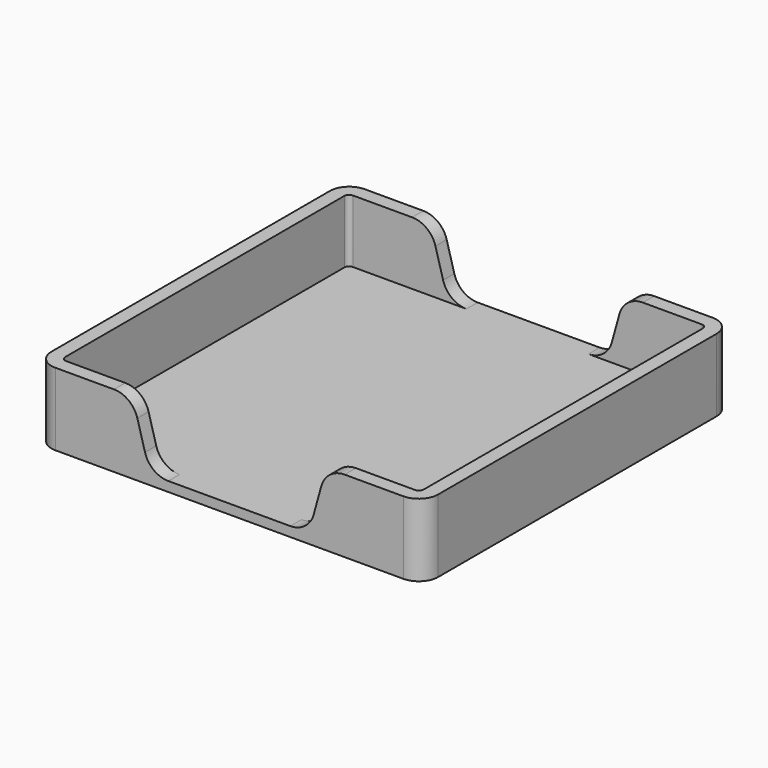
from build123d import *

# Parameters (mm, degrees)
F0_W      = 79.8
F0_H      = 79.8
F1_DEPTH  = 15
F2_W      = 74
F2_H      = 74
F3_DEPTH  = 13
F4_W      = 73.8
F4_H      = 73.8
F4_W_2    = 69.8
F4_H_2    = 69.8
F5_DEPTH  = 2
F7_DEPTH  = 2
F8_R      = 2
F9_R      = 4
F10_R     = 0.99999
F12_DEPTH = 79.801
F13_R     = 5
F14_R     = 4
F15_R     = 1


# Not quite as in the source:
# - a fillet or chamfer is up to 0.001 mm smaller than in the source, because OpenCascade refuses the exact size


with BuildPart() as f1:
    # F0 (on Top) → F1 (new body)
    with BuildSketch(Plane.XY):
        Rectangle(F0_W, F0_H)
    extrude(amount=F1_DEPTH)

    # F2 (on face) → F3 (cut)
    with BuildSketch(Plane.XY.offset(15)):
        Rectangle(F2_W, F2_H)
    extrude(amount=-F3_DEPTH, mode=Mode.SUBTRACT)

    # F4 (on face) → F5 (join)
    with BuildSketch(Plane(origin=(0, 0, 0), x_dir=(1, 0, 0), z_dir=(0, 0, -1))):
        Rectangle(F4_W, F4_H)
        Rectangle(F4_W_2, F4_H_2, mode=Mode.SUBTRACT)
    extrude(amount=F5_DEPTH)

    # F6 (on face) → F7 (cut, through all)
    with BuildSketch(Plane(origin=(0, 0, -2), x_dir=(1, 0, 0), z_dir=(0, 0, -1))):
        Polygon((36.9, -21.9), (36.9, 21.9), (21.9, 21.9), (21.9, 36.9), (-21.9, 36.9), (-21.9, 21.9), (-36.9, 21.9), (-36.9, -21.9), (-21.9, -21.9), (-21.9, -36.9), (21.9, -36.9), (21.9, -21.9), align=None)
    extrude(amount=-F7_DEPTH, mode=Mode.SUBTRACT)

    # F8
    f8_edges = [f1.edges().sort_by_distance(p)[0] for p in [
        (-34.9, 34.9, -1),
        (-34.9, -34.9, -1),
        (34.9, -34.9, -1),
        (34.9, 34.9, -1),
    ]]
    fillet(f8_edges, radius=F8_R)

    # F9
    f9_edges = [f1.edges().sort_by_distance(p)[0] for p in [
        (-36.9, 36.9, -1),
        (36.9, 36.9, -1),
        (36.9, -36.9, -1),
        (-36.9, -36.9, -1),
    ]]
    fillet(f9_edges, radius=F9_R)

    # F10 (radius 1 in the source; OpenCascade refuses exactly that, so slightly less here)
    f10_edges = [f1.edges().sort_by_distance(p)[0] for p in [
        (21.9, -35.9, -2),
        (21.9, -35.9, 0),
        (35.9, -21.9, -2),
        (35.9, -21.9, 0),
        (-35.9, -21.9, -2),
        (-35.9, -21.9, 0),
        (-21.9, -35.9, -2),
        (-21.9, -35.9, 0),
        (-35.9, 21.9, -2),
        (-35.9, 21.9, 0),
        (-21.9, 35.9, -2),
        (-21.9, 35.9, 0),
        (21.9, 35.9, -2),
        (21.9, 35.9, 0),
        (35.9, 21.9, -2),
        (35.9, 21.9, 0),
    ]]
    fillet(f10_edges, radius=F10_R)

    # F11 (on face) → F12 (cut, through all)
    with BuildSketch(Plane.XZ.offset(39.9)):
        Polygon((20, 15), (-20, 15), (-16.3888888889, 2), (16.3888888889, 2), align=None)
    extrude(amount=-F12_DEPTH, mode=Mode.SUBTRACT)

    # F13
    f13_edges = [f1.edges().sort_by_distance(p)[0] for p in [
        (-20, -38.45, 15),
        (-16.388889, -38.45, 2),
        (16.388889, -38.45, 2),
        (20, -38.45, 15),
        (16.388889, 38.45, 2),
        (20, 38.45, 15),
        (-20, 38.45, 15),
        (-16.388889, 38.45, 2),
    ]]
    fillet(f13_edges, radius=F13_R)

    # F14
    f14_edges = [f1.edges().sort_by_distance(p)[0] for p in [
        (39.9, -39.9, 7.5),
        (39.9, 39.9, 7.5),
        (-39.9, -39.9, 7.5),
        (-39.9, 39.9, 7.5),
    ]]
    fillet(f14_edges, radius=F14_R)

    # F15
    f15_edges = [f1.edges().sort_by_distance(p)[0] for p in [
        (37, 37, 8.5),
        (-37, 37, 8.5),
        (-37, -37, 8.5),
        (37, -37, 8.5),
    ]]
    fillet(f15_edges, radius=F15_R)


solid = f1.part
